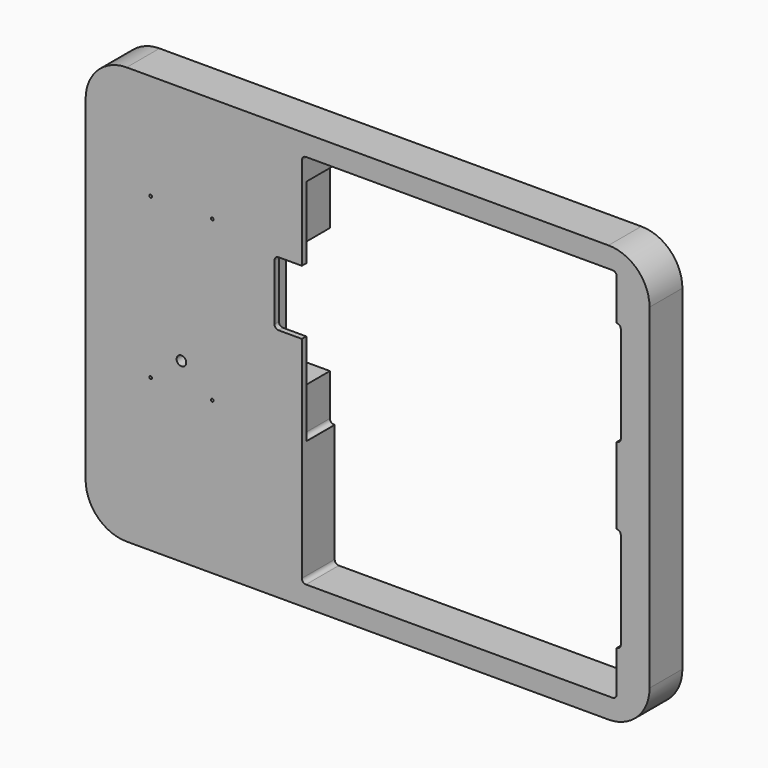
from build123d import *

# Parameters (mm, degrees)
F0_W      = 412
F0_H      = 305
F1_DEPTH  = 30
F2_W      = 230
F2_H      = 275
F3_DEPTH  = 30
F4_R      = 3
F5_R      = 30
F6_W      = 26
F6_H      = 167
F7_DEPTH  = 3.5
F8_R      = 3
F10_W     = 32
F10_H     = 92
F11_DEPTH = 26
F12_R     = 3
F13_W     = 4
F13_H     = 47
F14_DEPTH = 20
F15_R     = 3
F16_W     = 30
F16_H     = 76.5
F17_DEPTH = 3
F18_R     = 2.99999
F19_R     = 3.5
F20_DEPTH = 30
F21_W     = 99
F21_H     = 62
F22_DEPTH = 18
F23_R     = 3
F25_DEPTH = 6
F26_W     = 13
F26_H     = 20
F26_H_2   = 6
F27_DEPTH = 30
F28_R     = 1
F29_DEPTH = 30
F31_DEPTH = 20


# Not quite as in the source:
# - a fillet or chamfer is up to 0.001 mm smaller than in the source, because OpenCascade refuses the exact size
# - a feature names something its author has since deleted; it is built from what else it names


with BuildPart() as f1:
    # F0 (on Front) → F1 (new body)
    with BuildSketch(Plane.XZ):
        Rectangle(F0_W, F0_H)
    extrude(amount=F1_DEPTH)

    # F2 (on face) → F3 (cut, through all)
    with BuildSketch(Plane.XZ.offset(30)):
        with Locations((67, 0)):
            Rectangle(F2_W, F2_H)
    extrude(amount=-F3_DEPTH, mode=Mode.SUBTRACT)

    # F4
    f4_edges = [f1.edges().sort_by_distance(p)[0] for p in [
        (-48, -15, 137.5),
        (182, -15, 137.5),
        (182, -15, -137.5),
        (-48, -15, -137.5),
    ]]
    fillet(f4_edges, radius=F4_R)

    # F5
    f5_edges = [f1.edges().sort_by_distance(p)[0] for p in [
        (-206, -15, -152.5),
        (-206, -15, 152.5),
        (206, -15, 152.5),
        (206, -15, -152.5),
    ]]
    fillet(f5_edges, radius=F5_R)

    # F6 (on face) → F7 (cut)
    with BuildSketch(Plane.YZ.offset(-48)):
        with Locations((-13, 35.5)):
            Rectangle(F6_W, F6_H)
    extrude(amount=-F7_DEPTH, mode=Mode.SUBTRACT)

    # F8
    f8_edges = [f1.edges().sort_by_distance(p)[0] for p in [
        (-51.5, -13, -48),
        (-51.5, -13, 119),
    ]]
    fillet(f8_edges, radius=F8_R)

    # F10 (on face) → F11 (cut)
    with BuildSketch(Plane(origin=(0, 0, 0), x_dir=(-1, 0, 0), z_dir=(0, 1, 0))):
        with Locations((67.5, 31.5)):
            Rectangle(F10_W, F10_H)
    extrude(amount=-F11_DEPTH, mode=Mode.SUBTRACT)

    # F12
    f12_edges = [f1.edges().sort_by_distance(p)[0] for p in [
        (-83.5, -13, -14.5),
        (-83.5, -13, 77.5),
    ]]
    fillet(f12_edges, radius=F12_R)

    # F13 (on face) → F14 (cut)
    with BuildSketch(Plane.YZ.offset(-48)):
        with Locations((-28, 43)):
            Rectangle(F13_W, F13_H)
    extrude(amount=-F14_DEPTH, mode=Mode.SUBTRACT)

    # F15
    f15_edges = [f1.edges().sort_by_distance(p)[0] for p in [
        (-68, -28, 19.5),
        (-68, -28, 66.5),
    ]]
    fillet(f15_edges, radius=F15_R)

    # F16 (on face) → F17 (cut)
    with BuildSketch(Plane(origin=(182, 0, 0), x_dir=(0, -1, 0), z_dir=(-1, 0, 0))):
        with Locations((15, -66.25)):
            Rectangle(F16_W, F16_H)
        with Locations((15, 66.25)):
            Rectangle(F16_W, F16_H)
    extrude(amount=-F17_DEPTH, mode=Mode.SUBTRACT)

    # F18 (radius 3 in the source; OpenCascade refuses exactly that, so slightly less here)
    f18_edges = [f1.edges().sort_by_distance(p)[0] for p in [
        (185, -15, -104.5),
        (185, -15, 28),
        (185, -15, 104.5),
        (185, -15, -28),
    ]]
    fillet(f18_edges, radius=F18_R)

    # F19 (on face) → F20 (cut)
    with BuildSketch(Plane.XZ.offset(30)):
        with Locations((-136, -23.25)):
            Circle(F19_R)
    extrude(amount=-F20_DEPTH, mode=Mode.SUBTRACT)

    # F21 (on face) → F22 (cut)
    with BuildSketch(Plane(origin=(0, 0, 0), x_dir=(-1, 0, 0), z_dir=(0, 1, 0))):
        with Locations((126.5, -97.75)):
            Rectangle(F21_W, F21_H)
    extrude(amount=-F22_DEPTH, mode=Mode.SUBTRACT)

    # F23
    f23_edges = [f1.edges().sort_by_distance(p)[0] for p in [
        (-176, -9, -128.75),
        (-77, -9, -128.75),
        (-77, -9, -66.75),
        (-176, -9, -66.75),
    ]]
    fillet(f23_edges, radius=F23_R)

    # F24 (on face) → F25 (cut)
    with BuildSketch(Plane(origin=(0, 0, 0), x_dir=(-1, 0, 0), z_dir=(0, 1, 0))):
        with BuildLine():
            ThreePointArc((139.5, -23.25), (136, -26.75), (132.5, -23.25))
            Line((132.5, -23.25), (132.5, -66.75))
            Line((132.5, -66.75), (139.5, -66.75))
            Line((139.5, -66.75), (139.5, -23.25))
        make_face()
    extrude(amount=-F25_DEPTH, mode=Mode.SUBTRACT)

    # F26 (on face) → F27 (cut)
    with BuildSketch(Plane(origin=(-206, 0, 0), x_dir=(0, -1, 0), z_dir=(-1, 0, 0))):
        with Locations((6.5, -92.5)):
            Rectangle(F26_W, F26_H)
        with Locations((6.5, -113.5)):
            Rectangle(F26_W, F26_H_2)
    extrude(amount=-F27_DEPTH, mode=Mode.SUBTRACT)

    # F28 (on face) → F29 (cut)
    with BuildSketch(Plane.XZ.offset(30)):
        with Locations((-158.5, 75.35)):
            Circle(F28_R)
        with Locations((-158.5, -41.25)):
            Circle(F28_R)
        with Locations((-113.5, -41.25)):
            Circle(F28_R)
        with Locations((-113.5, 75.35)):
            Circle(F28_R)
    extrude(amount=-F29_DEPTH, mode=Mode.SUBTRACT)

    # F30 (on face) → F31 (cut)
    with BuildSketch(Plane(origin=(0, 0, 0), x_dir=(-1, 0, 0), z_dir=(0, 1, 0))):
        with BuildLine():
            Line((-194, 120), (-194, 122))
            ThreePointArc((-194, 122), (-195, 121), (-194, 120))
        make_face()
        with BuildLine():
            ThreePointArc((-193, 121), (-193.2928932188, 121.7071067812), (-194, 122))
            Line((-194, 122), (-194, 120))
            ThreePointArc((-194, 120), (-193.2928932188, 120.2928932188), (-193, 121))
        make_face()
        with BuildLine():
            ThreePointArc((-68, 145), (-67, 144), (-66, 145))
            Line((-66, 145), (-68, 145))
        make_face()
        with BuildLine():
            Line((-68, 145), (-66, 145))
            ThreePointArc((-66, 145), (-67, 146), (-68, 145))
        make_face()
        with BuildLine():
            Line((131.5, 145), (133.5, 145))
            ThreePointArc((133.5, 145), (132.5, 146), (131.5, 145))
        make_face()
        with BuildLine():
            ThreePointArc((131.5, 145), (132.5, 144), (133.5, 145))
            Line((133.5, 145), (131.5, 145))
        make_face()
        with BuildLine():
            ThreePointArc((192, 0), (191.7071067812, 0.7071067812), (191, 1))
            Line((191, 1), (191, -1))
            ThreePointArc((191, -1), (191.7071067812, -0.7071067812), (192, 0))
        make_face()
        with BuildLine():
            Line((191, -1), (191, 1))
            ThreePointArc((191, 1), (190, 0), (191, -1))
        make_face()
        with BuildLine():
            Line((131.5, -145), (133.5, -145))
            ThreePointArc((133.5, -145), (132.5, -144), (131.5, -145))
        make_face()
        with BuildLine():
            ThreePointArc((131.5, -145), (132.5, -146), (133.5, -145))
            Line((133.5, -145), (131.5, -145))
        make_face()
        with BuildLine():
            Line((-68, -145), (-66, -145))
            ThreePointArc((-66, -145), (-67, -144), (-68, -145))
        make_face()
        with BuildLine():
            ThreePointArc((-68, -145), (-67, -146), (-66, -145))
            Line((-66, -145), (-68, -145))
        make_face()
        with BuildLine():
            ThreePointArc((-193, -121), (-193.2928932188, -120.2928932188), (-194, -120))
            Line((-194, -120), (-194, -122))
            ThreePointArc((-194, -122), (-193.2928932188, -121.7071067812), (-193, -121))
        make_face()
        with BuildLine():
            Line((-194, -122), (-194, -120))
            ThreePointArc((-194, -120), (-195, -121), (-194, -122))
        make_face()
        with BuildLine():
            Line((-194, -1), (-194, 1))
            ThreePointArc((-194, 1), (-195, 0), (-194, -1))
        make_face()
        with BuildLine():
            ThreePointArc((-193, 0), (-193.2928932188, 0.7071067812), (-194, 1))
            Line((-194, 1), (-194, -1))
            ThreePointArc((-194, -1), (-193.2928932188, -0.7071067812), (-193, 0))
        make_face()
    extrude(amount=-F31_DEPTH, mode=Mode.SUBTRACT)


solid = f1.part
